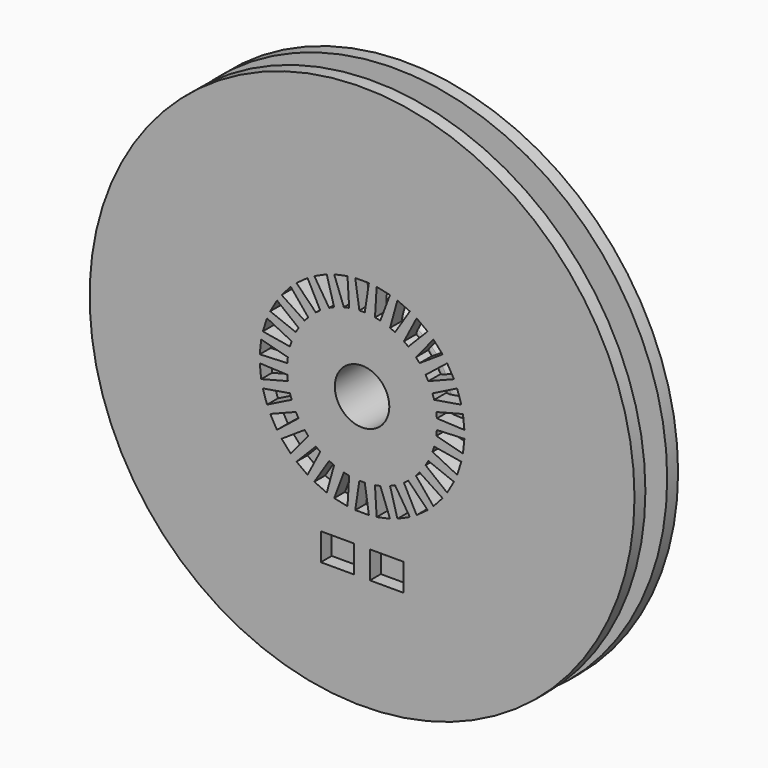
from build123d import *

# Parameters (mm, degrees)
F0_R            = 20
F0_R_2          = 2
F1_DEPTH        = 2
F4_W            = 2.4523979519
F4_H            = 2.005261369
F5_DEPTH        = 4.001
F6_DEPTH        = 4.001
F6_COPIES_COUNT = 30


# Not quite as in the source:
# - a pattern or mirror of a feature is missing from the dataset's text; its kind, count and spacing are read off the source's solid


with BuildPart() as f1:
    # F0 (on Front) → F1 (new body, symmetric)
    with BuildSketch(Plane.XZ):
        Circle(F0_R)
        Circle(F0_R_2, mode=Mode.SUBTRACT)
    extrude(amount=F1_DEPTH, both=True)

    # F2 (on Right) → F3 (revolve, cut)
    with BuildSketch(Plane.YZ):
        with BuildLine():
            Line((1, 20), (-1, 20))
            Line((-1, 20), (-1, 6))
            ThreePointArc((-1, 6), (0, 7), (1, 6))
            Line((1, 6), (1, 20))
        make_face()
        with BuildLine():
            ThreePointArc((1, 6), (0, 7), (-1, 6))
            ThreePointArc((-1, 6), (-0.7071067812, 5.2928932188), (0, 5))
            ThreePointArc((0, 5), (0.7071067812, 5.2928932188), (1, 6))
        make_face()
    revolve(axis=Axis((0, -2, 0), (0, -1, 0)), mode=Mode.SUBTRACT)

    # F4 (on face) → F5 (cut, through all)
    with BuildSketch(Plane.XZ.offset(2)):
        with Locations((-1.8047353951, -10.690020863)):
            Rectangle(F4_W, F4_H)
        with Locations((1.8047353951, -10.690020863)):
            Rectangle(F4_W, F4_H)
    extrude(amount=-F5_DEPTH, mode=Mode.SUBTRACT)

    # F4 (on face) → F6 (cut, through all)
    with BuildSketch(Plane.XZ.offset(2)):
        Polygon((0.2, -5.5), (0, -5.5), (-0.2, -5.5), (-0.5, -7.5), (0, -7.5), (0.5, -7.5), align=None)
    f6 = extrude(amount=-F6_DEPTH, mode=Mode.SUBTRACT)

    # F6_copies: F6 ×30 about axis
    f6_copies_axis = Axis((0, 0, 0), (0, 1, 0))
    for i in range(1, F6_COPIES_COUNT):
        add(f6.rotate(f6_copies_axis, i * 360 / F6_COPIES_COUNT), mode=Mode.SUBTRACT)


solid = f1.part
